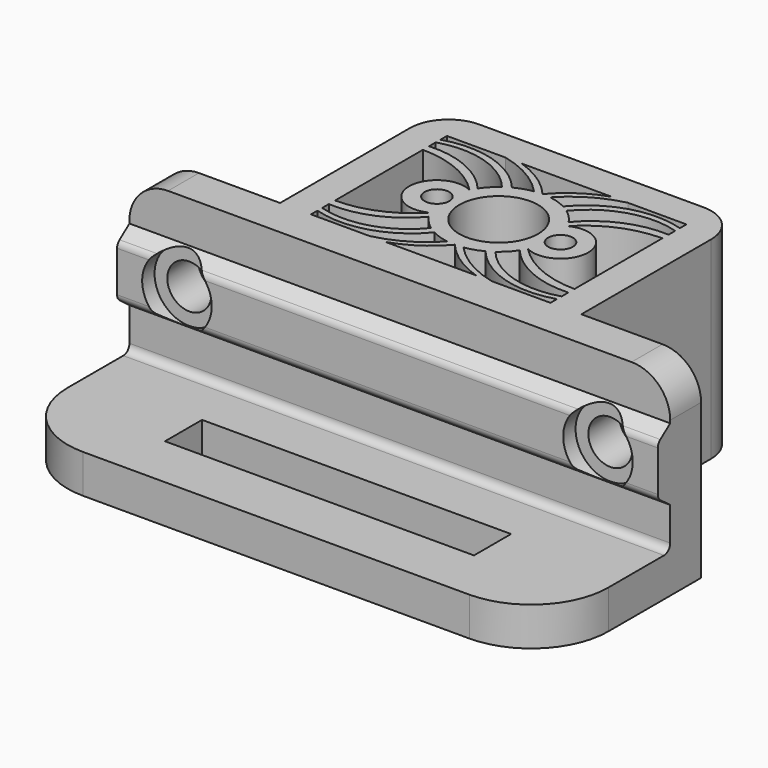
from build123d import *

# Parameters (mm, degrees)
F0_W     = 15
F0_H     = 5
F0_W_2   = 40
F0_H_2   = 7
F0_R     = 1.6
F0_R_2   = 5.1
F1_DEPTH = 25
F2_DEPTH = 20
F5_DEPTH = 70
F3_R     = 2.85
F6_DEPTH = 25.001
F7_R     = 4.5
F7_R_2   = 2.85
F8_DEPTH = 2
F9_R     = 5
F10_R    = 1


# Not quite as in the source:
# - ends of sketch curves that miss each other by under 0.0002 mm in the source are joined
# - a feature names something its author has since deleted; it is built from what else it names


with BuildPart() as f1:
    # F0 (on Top) → F1 (new body)
    with BuildSketch(Plane.XY):
        with Locations((-47.5, -7.1279055323)):
            Rectangle(F0_W, F0_H)
        with Locations((7.5, -7.1279055323)):
            Rectangle(F0_W, F0_H)
        with Locations((-20, -26.1279055323)):
            Rectangle(F0_W_2, F0_H_2)
        with BuildLine():
            ThreePointArc((-13.6593749135, 9.5668516592), (-9.4804951392, 12.4620627067), (-4.5000003888, 13.481844654))
            Line((-4.5000003888, 13.481844654), (-4.5000003888, 14.481844654))
            ThreePointArc((-4.5000003888, 14.481844654), (-9.793949685, 13.5428339695), (-14.1101168945, 10.3368488111))
            ThreePointArc((-14.1101168945, 10.3368488111), (-13.872638695, 9.9589375697), (-13.6593749135, 9.5668516592))
        make_face()
        with BuildLine():
            ThreePointArc((-15.8291388207, 12.1178683079), (-10.6891300848, 15.5654287884), (-4.5000003888, 15.5593724921))
            Line((-4.5000003888, 15.5593724921), (-4.5000003888, 16.3141830726))
            ThreePointArc((-4.5000003888, 16.3141830726), (-11.1501915503, 16.3321080887), (-16.6903423933, 12.6535088408))
            ThreePointArc((-16.6903423933, 12.6535088408), (-16.2501642673, 12.4010854262), (-15.8291388207, 12.1178683079))
        make_face()
        with BuildLine():
            ThreePointArc((-18.9549587768, 13.3947641055), (-15.8181752362, 15.9024378017), (-12.0808034818, 17.3720944677))
            Line((-12.0808034818, 17.3720944677), (-14.1525114111, 17.3720944677))
            ThreePointArc((-14.1525114111, 17.3720944677), (-17.3497652419, 15.8321825785), (-20.0000000983, 13.4720944677))
            ThreePointArc((-20, 13.4720944677), (-19.4760507794, 13.4527354849), (-18.9549587768, 13.3947641055))
        make_face()
        with BuildLine():
            Line((-25.8474885889, 17.3720944677), (-27.9191965182, 17.3720944677))
            ThreePointArc((-27.9191965182, 17.3720944677), (-24.1818247638, 15.9024378017), (-21.0450412232, 13.3947641055))
            ThreePointArc((-21.0450412232, 13.3947641055), (-20.5239492206, 13.4527354849), (-20, 13.4720944677))
            ThreePointArc((-19.9999999017, 13.4720944677), (-22.6502347581, 15.8321825785), (-25.8474885889, 17.3720944677))
        make_face()
        with BuildLine():
            Line((-35.4999996112, 16.3141830726), (-35.4999996112, 15.5593724921))
            ThreePointArc((-35.4999996112, 15.5593724921), (-29.3108699152, 15.5654287884), (-24.1708611793, 12.1178683079))
            ThreePointArc((-24.1708611793, 12.1178683079), (-23.7498357327, 12.4010854262), (-23.3096576067, 12.6535088408))
            ThreePointArc((-23.3096576067, 12.6535088408), (-28.8498084497, 16.3321080887), (-35.4999996112, 16.3141830726))
        make_face()
        with BuildLine():
            Line((-35.4999996112, 14.481844654), (-35.4999996112, 13.481844654))
            ThreePointArc((-35.4999996112, 13.481844654), (-30.5195048608, 12.4620627067), (-26.3406250865, 9.5668516592))
            ThreePointArc((-26.3406250865, 9.5668516592), (-26.1273613547, 9.9589374848), (-25.8898831055, 10.3368488111))
            ThreePointArc((-25.8898831055, 10.3368488111), (-30.206050315, 13.5428339695), (-35.4999996112, 14.481844654))
        make_face()
        with BuildLine():
            Line((-35.4999996112, -0.7376557186), (-35.4999996112, -1.7376557186))
            ThreePointArc((-35.4999996112, -1.7376557186), (-30.206050315, -0.7986450341), (-25.8898831055, 2.4073401243))
            ThreePointArc((-25.8898831055, 2.4073401243), (-26.1273613547, 2.7852514506), (-26.340625175, 3.1773374518))
            ThreePointArc((-26.340625175, 3.1773374518), (-30.5195048608, 0.2821262287), (-35.4999996112, -0.7376557186))
        make_face()
        with BuildLine():
            Line((-35.4999996112, -2.8151835567), (-35.4999996112, -3.5699941372))
            ThreePointArc((-35.4999996112, -3.5699941372), (-28.8498084497, -3.5879191533), (-23.3096576067, 0.0906800946))
            ThreePointArc((-23.3096576067, 0.0906800946), (-23.7498357327, 0.3431035092), (-24.1708611793, 0.6263206275))
            ThreePointArc((-24.1708611793, 0.6263206275), (-29.3108699152, -2.821239853), (-35.4999996112, -2.8151835567))
        make_face()
        with BuildLine():
            ThreePointArc((-16.6903423933, 0.0906800946), (-11.1501915503, -3.5879191533), (-4.5000003888, -3.5699941372))
            Line((-4.5000003888, -3.5699941372), (-4.5000003888, -2.8151835567))
            ThreePointArc((-4.5000003888, -2.8151835567), (-10.6891300848, -2.821239853), (-15.8291388207, 0.6263206275))
            ThreePointArc((-15.8291388207, 0.6263206275), (-16.2501642673, 0.3431035092), (-16.6903423933, 0.0906800946))
        make_face()
        with BuildLine():
            ThreePointArc((-14.1101168945, 2.4073401243), (-9.793949685, -0.7986450341), (-4.5000003888, -1.7376557186))
            Line((-4.5000003888, -1.7376557186), (-4.5000003888, -0.7376557186))
            ThreePointArc((-4.5000003888, -0.7376557186), (-9.4804951392, 0.2821262287), (-13.6593749135, 3.1773372762))
            ThreePointArc((-13.6593749135, 3.1773372762), (-13.872638695, 2.7852513658), (-14.1101168945, 2.4073401243))
        make_face()
        with BuildLine():
            Line((-45, -29.6279055323), (-40, -29.6279055323))
            Line((-40, -29.6279055323), (-40, -22.6279055323))
            Line((-40, -22.6279055323), (-40, -16.6279055323))
            Line((-40, -16.6279055323), (-40, -9.6279055323))
            Line((-40, -9.6279055323), (-55, -9.6279055323))
            Line((-55, -9.6279055323), (-55, -19.6279055323))
            ThreePointArc((-55, -19.6279055323), (-52.0710678119, -26.6989733442), (-45, -29.6279055323))
        make_face()
        with BuildLine():
            Line((0, -22.6279055323), (0, -29.6279055323))
            Line((0, -29.6279055323), (5, -29.6279055323))
            ThreePointArc((5, -29.6279055323), (12.0710678119, -26.6989733442), (15, -19.6279055323))
            Line((15, -19.6279055323), (15, -9.6279055323))
            Line((15, -9.6279055323), (0, -9.6279055323))
            Line((0, -9.6279055323), (0, -16.6279055323))
            Line((0, -16.6279055323), (0, -22.6279055323))
        make_face()
        Polygon((-40, -4.6279055323), (-40, -9.6279055323), (0, -9.6279055323), (0, -4.6279055323), (-0.5000019073, -4.6279055323), (-4.5000003888, -4.6279055323), (-12.0808034818, -4.6279055323), (-14.1525114111, -4.6279055323), (-25.8474885889, -4.6279055323), (-27.9191965182, -4.6279055323), (-35.4999996112, -4.6279055323), (-39.4999980927, -4.6279055323), align=None)
        with BuildLine():
            ThreePointArc((-23.3096576067, 0.0906800946), (-22.2086682224, -0.3756299401), (-21.0450412232, -0.6505751701))
            ThreePointArc((-21.0450412232, -0.6505751701), (-20.5239492206, -0.7085465495), (-20, -0.7279055323))
            ThreePointArc((-20, -0.7279055323), (-19.4760507794, -0.7085465495), (-18.9549587768, -0.6505751701))
            ThreePointArc((-18.9549587768, -0.6505751701), (-17.7913317776, -0.3756299401), (-16.6903423933, 0.0906800946))
            ThreePointArc((-16.6903423933, 0.0906800946), (-16.2501642673, 0.3431035092), (-15.8291388207, 0.6263206275))
            ThreePointArc((-15.8291388207, 0.6263206275), (-14.8914139429, 1.4413390999), (-14.1101168945, 2.4073401243))
            ThreePointArc((-14.1101168945, 2.4073401243), (-13.872638695, 2.7852513658), (-13.6593749135, 3.1773372762))
            ThreePointArc((-13.6593749135, 3.1773372762), (-8.4000001922, 6.3720944677), (-13.6593749135, 9.5668516592))
            ThreePointArc((-13.6593749135, 9.5668516592), (-13.872638695, 9.9589375697), (-14.1101168945, 10.3368488111))
            ThreePointArc((-14.1101168945, 10.3368488111), (-14.8914139429, 11.3028498355), (-15.8291388207, 12.1178683079))
            ThreePointArc((-15.8291388207, 12.1178683079), (-16.2501642673, 12.4010854262), (-16.6903423933, 12.6535088408))
            ThreePointArc((-16.6903423933, 12.6535088408), (-17.7913317776, 13.1198188755), (-18.9549587768, 13.3947641055))
            ThreePointArc((-18.9549587768, 13.3947641055), (-19.4760507794, 13.4527354849), (-20, 13.4720944677))
            ThreePointArc((-20, 13.4720944677), (-20.5239492206, 13.4527354849), (-21.0450412232, 13.3947641055))
            ThreePointArc((-21.0450412232, 13.3947641055), (-22.2086682224, 13.1198188755), (-23.3096576067, 12.6535088408))
            ThreePointArc((-23.3096576067, 12.6535088408), (-23.7498357327, 12.4010854262), (-24.1708611793, 12.1178683079))
            ThreePointArc((-24.1708611793, 12.1178683079), (-25.1085860571, 11.3028498355), (-25.8898831055, 10.3368488111))
            ThreePointArc((-25.8898831055, 10.3368488111), (-26.1273613547, 9.9589374848), (-26.340625175, 9.5668514836))
            ThreePointArc((-26.340625175, 9.5668514836), (-31.5999996112, 6.3720944677), (-26.340625175, 3.1773374518))
            ThreePointArc((-26.340625175, 3.1773374518), (-26.1273613547, 2.7852514506), (-25.8898831055, 2.4073401243))
            ThreePointArc((-25.8898831055, 2.4073401243), (-25.1085860571, 1.4413390999), (-24.1708611793, 0.6263206275))
            ThreePointArc((-24.1708611793, 0.6263206275), (-23.7498357327, 0.3431035092), (-23.3096576067, 0.0906800946))
        make_face()
        with Locations((-28, 6.3720944677)):
            Circle(F0_R, mode=Mode.SUBTRACT)
        with Locations((-20, 6.3720944677)):
            Circle(F0_R_2, mode=Mode.SUBTRACT)
        with Locations((-12, 6.3720944677)):
            Circle(F0_R, mode=Mode.SUBTRACT)
        with BuildLine():
            Line((-14.1525114111, -4.6279055323), (-12.0808034818, -4.6279055323))
            ThreePointArc((-12.0808034818, -4.6279055323), (-15.8181752362, -3.1582488663), (-18.9549587768, -0.6505751701))
            ThreePointArc((-18.9549587768, -0.6505751701), (-19.4760507794, -0.7085465495), (-20, -0.7279055323))
            ThreePointArc((-20.0000000983, -0.7279055323), (-17.3497652419, -3.0879936431), (-14.1525114111, -4.6279055323))
        make_face()
        with BuildLine():
            ThreePointArc((-21.0450412232, -0.6505751701), (-24.1818247638, -3.1582488663), (-27.9191965182, -4.6279055323))
            Line((-27.9191965182, -4.6279055323), (-25.8474885889, -4.6279055323))
            ThreePointArc((-25.8474885889, -4.6279055323), (-22.6502347581, -3.0879936431), (-19.9999999017, -0.7279055323))
            ThreePointArc((-20, -0.7279055323), (-20.5239492206, -0.7085465495), (-21.0450412232, -0.6505751701))
        make_face()
        with BuildLine():
            Line((-39.4999980927, 16.3720929492), (-39.4999980927, -4.6279055323))
            Line((-39.4999980927, -4.6279055323), (-35.4999996112, -4.6279055323))
            Line((-35.4999996112, -4.6279055323), (-35.4999996112, -3.5699941372))
            Line((-35.4999996112, -3.5699941372), (-35.4999996112, -2.8151835567))
            Line((-35.4999996112, -2.8151835567), (-35.4999996112, -1.7376557186))
            Line((-35.4999996112, -1.7376557186), (-35.4999996112, -0.7376557186))
            Line((-35.4999996112, -0.7376557186), (-35.4999996112, 13.481844654))
            Line((-35.4999996112, 13.481844654), (-35.4999996112, 14.481844654))
            Line((-35.4999996112, 14.481844654), (-35.4999996112, 15.5593724921))
            Line((-35.4999996112, 15.5593724921), (-35.4999996112, 16.3141830726))
            Line((-35.4999996112, 16.3141830726), (-35.4999996112, 17.3720944677))
            Line((-35.4999996112, 17.3720944677), (-27.9191965182, 17.3720944677))
            Line((-27.9191965182, 17.3720944677), (-25.8474885889, 17.3720944677))
            Line((-25.8474885889, 17.3720944677), (-14.1525114111, 17.3720944677))
            Line((-14.1525114111, 17.3720944677), (-12.0808034818, 17.3720944677))
            Line((-12.0808034818, 17.3720944677), (-4.5000003888, 17.3720944677))
            Line((-4.5000003888, 17.3720944677), (-4.5000003888, 16.3141830726))
            Line((-4.5000003888, 16.3141830726), (-4.5000003888, 15.5593724921))
            Line((-4.5000003888, 15.5593724921), (-4.5000003888, 14.481844654))
            Line((-4.5000003888, 14.481844654), (-4.5000003888, 13.481844654))
            Line((-4.5000003888, 13.481844654), (-4.5000003888, -0.7376557186))
            Line((-4.5000003888, -0.7376557186), (-4.5000003888, -1.7376557186))
            Line((-4.5000003888, -1.7376557186), (-4.5000003888, -2.8151835567))
            Line((-4.5000003888, -2.8151835567), (-4.5000003888, -3.5699941372))
            Line((-4.5000003888, -3.5699941372), (-4.5000003888, -4.6279055323))
            Line((-4.5000003888, -4.6279055323), (-0.5000019073, -4.6279055323))
            Line((-0.5000019073, -4.6279055323), (-0.5000019073, 16.3720929492))
            ThreePointArc((-0.5000019073, 16.3720929492), (-1.9644680014, 19.9076268551), (-5.5000019073, 21.3720929492))
            Line((-5.5000019073, 21.3720929492), (-34.4999980927, 21.3720929492))
            ThreePointArc((-34.4999980927, 21.3720929492), (-38.0355319986, 19.9076268551), (-39.4999980927, 16.3720929492))
        make_face()
        with Locations((-20, -13.1279055323)):
            Rectangle(F0_W_2, F0_H_2)
    extrude(amount=-F1_DEPTH)

    # F0 (on Top) → F2 (cut)
    with BuildSketch(Plane.XY):
        with Locations((-20, -26.1279055323)):
            Rectangle(F0_W_2, F0_H_2)
        with BuildLine():
            Line((-45, -29.6279055323), (-40, -29.6279055323))
            Line((-40, -29.6279055323), (-40, -22.6279055323))
            Line((-40, -22.6279055323), (-40, -16.6279055323))
            Line((-40, -16.6279055323), (-40, -9.6279055323))
            Line((-40, -9.6279055323), (-55, -9.6279055323))
            Line((-55, -9.6279055323), (-55, -19.6279055323))
            ThreePointArc((-55, -19.6279055323), (-52.0710678119, -26.6989733442), (-45, -29.6279055323))
        make_face()
        with BuildLine():
            Line((0, -22.6279055323), (0, -29.6279055323))
            Line((0, -29.6279055323), (5, -29.6279055323))
            ThreePointArc((5, -29.6279055323), (12.0710678119, -26.6989733442), (15, -19.6279055323))
            Line((15, -19.6279055323), (15, -9.6279055323))
            Line((15, -9.6279055323), (0, -9.6279055323))
            Line((0, -9.6279055323), (0, -16.6279055323))
            Line((0, -16.6279055323), (0, -22.6279055323))
        make_face()
        with Locations((-20, -13.1279055323)):
            Rectangle(F0_W_2, F0_H_2)
    extrude(amount=-F2_DEPTH, mode=Mode.SUBTRACT)

    # F4 (on face) → F5 (join, through all)
    with BuildSketch(Plane.YZ.offset(15)):
        with BuildLine():
            Line((-11.6279055323, -7.35), (-11.6279055323, -10))
            Line((-11.6279055323, -10), (-11.6279055323, -12.65))
            ThreePointArc((-11.6279055323, -12.65), (-11.5223327233, -13.0972135955), (-11.2279055323, -13.45))
            Line((-11.2279055323, -13.45), (-9.6279055323, -14.65))
            Line((-9.6279055323, -14.65), (-9.6279055323, -10))
            Line((-9.6279055323, -10), (-9.6279055323, -5.35))
            Line((-9.6279055323, -5.35), (-11.2279055323, -6.55))
            ThreePointArc((-11.2279055323, -6.55), (-11.5223327233, -6.9027864045), (-11.6279055323, -7.35))
        make_face()
    extrude(amount=-F5_DEPTH)

    # F3 (on face) → F6 (cut, through all)
    with BuildSketch(Plane(origin=(0, -4.6279055323, 0), x_dir=(-1, 0, 0), z_dir=(0, 1, 0))):
        with Locations((47.2499990463, -10)):
            Circle(F3_R)
        with Locations((-7.2499990463, -10)):
            Circle(F3_R)
    extrude(amount=-F6_DEPTH, mode=Mode.SUBTRACT)

    # F7 (on face) → F8 (cut, through all)
    with BuildSketch(Plane.XZ.offset(11.6279055323)):
        with Locations((7.2499990463, -10)):
            Circle(F7_R)
        with Locations((7.2499990463, -10)):
            Circle(F7_R_2, mode=Mode.SUBTRACT)
        with Locations((-47.2499990463, -10)):
            Circle(F7_R)
    extrude(amount=-F8_DEPTH, mode=Mode.SUBTRACT)

    # F9
    f9_edges = [f1.edges().sort_by_distance(p)[0] for p in [
        (15, -7.127906, 0),
        (-55, -7.127906, 0),
    ]]
    fillet(f9_edges, radius=F9_R)

    # F10
    f10_edges = [f1.edges().sort_by_distance(p)[0] for p in [
        (-20, -9.627906, -20),
    ]]
    fillet(f10_edges, radius=F10_R)


solid = f1.part
